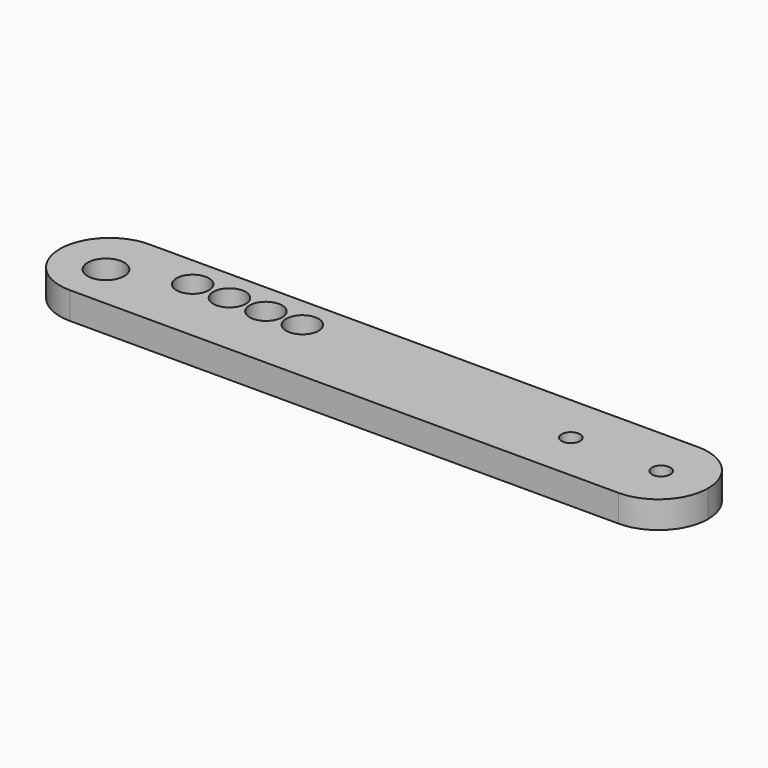
from build123d import *

# Parameters (mm, degrees)
F0_R     = 12.8905
F0_R_2   = 11.43
F0_R_3   = 6.5405
F1_DEPTH = 19.05
F2_R     = 34.92499


# Not quite as in the source:
# - a fillet or chamfer is up to 0.001 mm smaller than in the source, because OpenCascade refuses the exact size


with BuildPart() as f1:
    # F0 (on Top) → F1 (new body)
    with BuildSketch(Plane.XY):
        with BuildLine():
            Line((421.005, 38.1), (0, 38.1))
            ThreePointArc((0, 38.1), (-34.925, 3.175), (0, -31.75))
            Line((0, -31.75), (421.005, -31.75))
            Line((421.005, -31.75), (421.005, 38.1))
        make_face()
        Circle(F0_R, mode=Mode.SUBTRACT)
        with Locations((48.26, 15.875)):
            Circle(F0_R_2, mode=Mode.SUBTRACT)
        with Locations((74.168, 15.875)):
            Circle(F0_R_2, mode=Mode.SUBTRACT)
        with Locations((99.822, 15.875)):
            Circle(F0_R_2, mode=Mode.SUBTRACT)
        with Locations((125.476, 15.875)):
            Circle(F0_R_2, mode=Mode.SUBTRACT)
        with Locations((324.485, 3.175)):
            Circle(F0_R_3, mode=Mode.SUBTRACT)
        with Locations((387.985, 3.175)):
            Circle(F0_R_3, mode=Mode.SUBTRACT)
    extrude(amount=F1_DEPTH)

    # F2 (radius 34.925 in the source; OpenCascade refuses exactly that, so slightly less here)
    f2_edges = [f1.edges().sort_by_distance(p)[0] for p in [
        (421.005, 38.1, 9.525),
        (421.005, -31.75, 9.525),
    ]]
    fillet(f2_edges, radius=F2_R)


solid = f1.part
